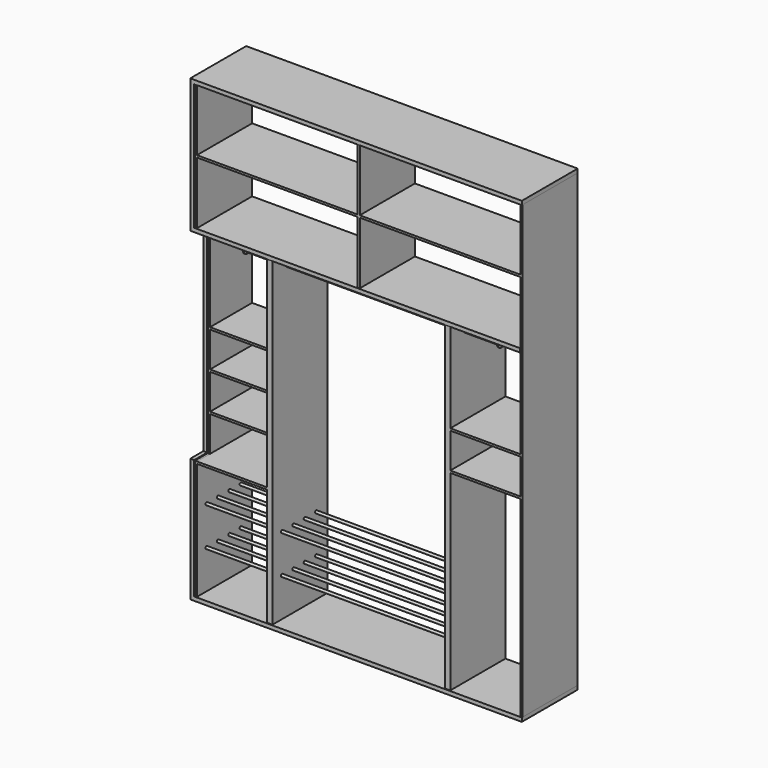
from build123d import *

# Parameters (mm, degrees)
F1_DEPTH       = 398
F0_W           = 30
F0_H           = 1828
F2_DEPTH       = 393
F0_W_2         = 12
F3_R           = 7.5
F4_DEPTH       = 1414
F5_W           = 400
F5_H           = 12
F6_DEPTH       = 393
F8_DEPTH       = 434
F9_DEPTH       = 5
F10_DEPTH      = 5
F11_R          = 15
F12_DEPTH      = 1214
F12_DEPTH_BACK = 230
F13_R          = 25
F13_R_2        = 15
F14_DEPTH      = 5
F15_R          = 25
F15_R_2        = 15
F16_DEPTH      = 5


with BuildPart() as f1:
    # F0 (on Front) → F1 (new body)
    with BuildSketch(Plane.XZ):
        Polygon((-1890, 0), (0, 0), (0, 22), (-12, 22), (-412, 22), (-442, 22), (-1426, 22), (-1456, 22), (-1856, 22), (-1868, 22), (-1868, 1850), (-1856, 1850), (-1456, 1850), (-1426, 1850), (-442, 1850), (-412, 1850), (-12, 1850), (-12, 1872), (-928, 1872), (-940, 1872), (-1856, 1872), (-1868, 1872), (-1868, 2593), (-1856, 2593), (-940, 2593), (-928, 2593), (-12, 2593), (0, 2593), (0, 2615), (-1890, 2615), align=None)
    extrude(amount=F1_DEPTH)


with BuildPart() as f2:
    # F0 (on Front) → F2 (new body, through all)
    with BuildSketch(Plane.XZ):
        with Locations((-1441, 936)):
            Rectangle(F0_W, F0_H)
    extrude(amount=F2_DEPTH)

    # F5 (on Front) → F6 (join, through all)
    with BuildSketch(Plane.XZ):
        with Locations((-1656, 1331.5)):
            Rectangle(F5_W, F5_H)
        with Locations((-1656, 1119.5)):
            Rectangle(F5_W, F5_H)
        with Locations((-1656, 907.5)):
            Rectangle(F5_W, F5_H)
        with Locations((-1656, 695.5)):
            Rectangle(F5_W, F5_H)
    extrude(amount=F6_DEPTH)


with BuildPart() as f2b:
    # F0 (on Front) → F2, piece 2 (new body, through all)
    with BuildSketch(Plane.XZ):
        with Locations((-427, 936)):
            Rectangle(F0_W, F0_H)
    extrude(amount=F2_DEPTH)


with BuildPart() as f2c:
    # F0 (on Front) → F2, piece 3 (new body, through all)
    with BuildSketch(Plane.XZ):
        Polygon((-12, 22), (0, 22), (0, 2593), (-12, 2593), (-12, 2238.5), (-928, 2238.5), (-928, 2593), (-940, 2593), (-940, 2238.5), (-1856, 2238.5), (-1856, 2593), (-1868, 2593), (-1868, 1872), (-1856, 1872), (-1856, 2226.5), (-940, 2226.5), (-940, 1872), (-928, 1872), (-928, 2226.5), (-12, 2226.5), (-12, 1872), (-12, 1850), align=None)
    extrude(amount=F2_DEPTH)


with BuildPart() as f2d:
    # F0 (on Front) → F2, piece 4 (new body, through all)
    with BuildSketch(Plane.XZ):
        with Locations((-1862, 936)):
            Rectangle(F0_W_2, F0_H)
    extrude(amount=F2_DEPTH)


with BuildPart() as f4:
    # F3 (on face) → F4 (new body, through all)
    with BuildSketch(Plane.YZ.offset(-1856)):
        with Locations((-324.5, 242)):
            Circle(F3_R)
    extrude(amount=F4_DEPTH)


with BuildPart() as f4b:
    # F3 (on face) → F4, piece 2 (new body, through all)
    with BuildSketch(Plane.YZ.offset(-1856)):
        with Locations((-324.5, 462)):
            Circle(F3_R)
    extrude(amount=F4_DEPTH)


with BuildPart() as f4c:
    # F3 (on face) → F4, piece 3 (new body, through all)
    with BuildSketch(Plane.YZ.offset(-1856)):
        with Locations((-243.5, 242)):
            Circle(F3_R)
    extrude(amount=F4_DEPTH)


with BuildPart() as f4d:
    # F3 (on face) → F4, piece 4 (new body, through all)
    with BuildSketch(Plane.YZ.offset(-1856)):
        with Locations((-243.5, 462)):
            Circle(F3_R)
    extrude(amount=F4_DEPTH)


with BuildPart() as f4e:
    # F3 (on face) → F4, piece 5 (new body, through all)
    with BuildSketch(Plane.YZ.offset(-1856)):
        with Locations((-162.5, 242)):
            Circle(F3_R)
    extrude(amount=F4_DEPTH)


with BuildPart() as f4f:
    # F3 (on face) → F4, piece 6 (new body, through all)
    with BuildSketch(Plane.YZ.offset(-1856)):
        with Locations((-162.5, 462)):
            Circle(F3_R)
    extrude(amount=F4_DEPTH)


with BuildPart() as f4g:
    # F3 (on face) → F4, piece 7 (new body, through all)
    with BuildSketch(Plane.YZ.offset(-1856)):
        with Locations((-81.5, 242)):
            Circle(F3_R)
    extrude(amount=F4_DEPTH)


with BuildPart() as f4h:
    # F3 (on face) → F4, piece 8 (new body, through all)
    with BuildSketch(Plane.YZ.offset(-1856)):
        with Locations((-81.5, 462)):
            Circle(F3_R)
    extrude(amount=F4_DEPTH)


with BuildPart() as f6:
    # F5 (on Front) → F6, piece 2 (new body, through all)
    with BuildSketch(Plane.XZ):
        with Locations((-212, 1331.5)):
            Rectangle(F5_W, F5_H)
    extrude(amount=F6_DEPTH)


with BuildPart() as f6b:
    # F5 (on Front) → F6, piece 3 (new body, through all)
    with BuildSketch(Plane.XZ):
        with Locations((-212, 1119.5)):
            Rectangle(F5_W, F5_H)
    extrude(amount=F6_DEPTH)


with BuildPart() as f8_tool:
    # F7 (on face) → F8 (new body, through all)
    with BuildSketch(Plane(origin=(-1890, 0, 0), x_dir=(0, -1, 0), z_dir=(-1, 0, 0))):
        Polygon((964.3889665604, 701.5), (976.9414663315, 1850), (300, 1850), (300, 701.5), align=None)
    extrude(amount=-F8_DEPTH)


with BuildPart() as f1_1:
    add(f1.part)

    # F8: cut by f8_tool
    add(f8_tool.part, mode=Mode.SUBTRACT)

    # F9 (add): a face of the model
    f9_faces = [f1_1.faces().sort_by_distance(p)[0] for p in [
        (-1879, -300, 1275.75),
    ]]
    extrude(f9_faces, amount=F9_DEPTH)

    # F10 (add): a face of the model
    f10_faces = [f1_1.faces().sort_by_distance(p)[0] for p in [
        (-1879, -351.5, 701.5),
    ]]
    extrude(f10_faces, amount=F10_DEPTH)


with BuildPart() as f2_1:
    add(f2.part)

    # F8: cut by f8_tool
    add(f8_tool.part, mode=Mode.SUBTRACT)


with BuildPart() as f2d_1:
    add(f2d.part)

    # F8: cut by f8_tool
    add(f8_tool.part, mode=Mode.SUBTRACT)


with BuildPart() as f12:
    # F11 (on face) → F12 (new body, two sides)
    with BuildSketch(Plane.YZ.offset(-1426)) as f12_sk:
        with Locations((-285, 1790)):
            Circle(F11_R)
    extrude(amount=F12_DEPTH)
    extrude(f12_sk.sketch, amount=-F12_DEPTH_BACK)


with BuildPart() as f14:
    # F13 (on face) → F14 (new body)
    with BuildSketch(Plane(origin=(-1656, 0, 0), x_dir=(0, -1, 0), z_dir=(-1, 0, 0))):
        with Locations((285, 1790)):
            Circle(F13_R)
        with Locations((285, 1790)):
            Circle(F13_R_2, mode=Mode.SUBTRACT)
        with Locations((285, 1790)):
            Circle(F13_R_2)
    extrude(amount=F14_DEPTH)


with BuildPart() as f16:
    # F15 (on face) → F16 (new body)
    with BuildSketch(Plane.YZ.offset(-212)):
        with Locations((-285, 1790)):
            Circle(F15_R)
        with Locations((-285, 1790)):
            Circle(F15_R_2, mode=Mode.SUBTRACT)
        with Locations((-285, 1790)):
            Circle(F15_R_2)
    extrude(amount=F16_DEPTH)


solid = Compound([f2b.part, f2c.part, f4.part, f4b.part, f4c.part, f4d.part, f4e.part, f4f.part, f4g.part, f4h.part, f6.part, f6b.part, f1_1.part, f2_1.part, f2d_1.part, f12.part, f14.part, f16.part])
